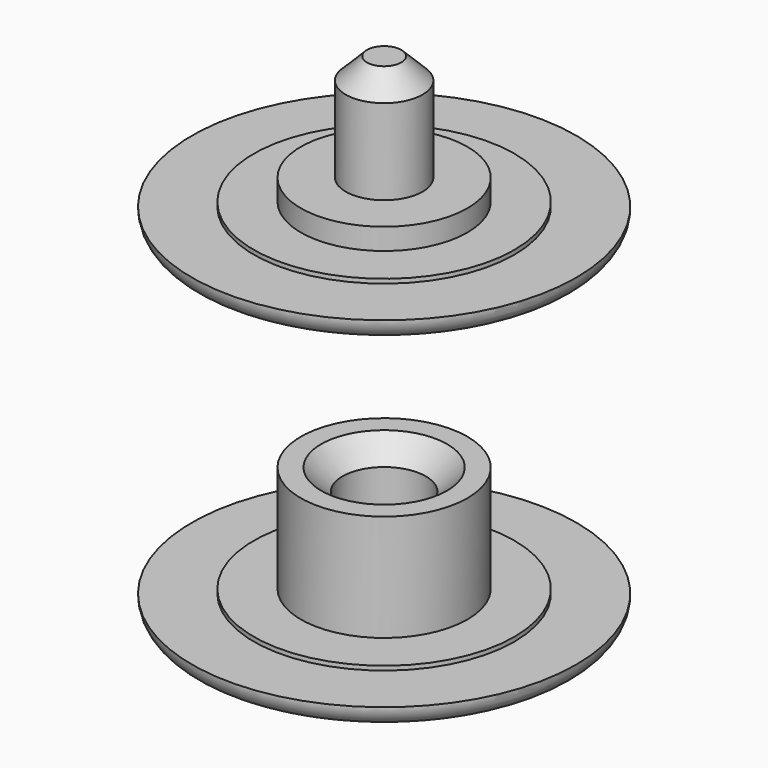
from build123d import *

# Parameters (mm, degrees)
F2_R    = 0.99999
F3_SIZE = 1
F6_R    = 0.99999
F7_SIZE = 1


# Not quite as in the source:
# - a fillet or chamfer is up to 0.001 mm smaller than in the source, because OpenCascade refuses the exact size


with BuildPart() as f1:
    # F0 (on Front) → F1 (revolve)
    with BuildSketch(Plane.XZ):
        Polygon((0, 1), (0, 0), (9, 0), (9, 1), (6.1, 1), (6.1, 1.2), (3.9, 1.2), (3.9, 6.2), (1.95, 6.2), (1.95, 2.2), (0, 2.2), (0, 1.7075754004), align=None)
    revolve(axis=Axis((0, 0, 1.9537877002), (0, 0, 1)))

    # F2 (radius 1 in the source; OpenCascade refuses exactly that, so slightly less here)
    f2_edges = [f1.edges().sort_by_distance(p)[0] for p in [
        (-9, 0, 0),
    ]]
    fillet(f2_edges, radius=F2_R)

    # F3
    f3_edges = [f1.edges().sort_by_distance(p)[0] for p in [
        (-1.95, 0, 6.2),
    ]]
    chamfer(f3_edges, length=F3_SIZE)


with BuildPart() as f5:
    # F4 (on Front) → F5 (revolve)
    with BuildSketch(Plane.XZ):
        Polygon((0, 16.9479211028), (0, 15.9479211028), (9, 15.9479211028), (9, 16.9479211028), (6.1, 16.9479211028), (6.1, 17.1479211028), (3.9, 17.1479211028), (3.9, 18.1479211028), (1.8, 18.1479211028), (1.8, 23.1479211028), (0, 23.1479211028), (0, 18.1479211028), (0, 17.1479211028), align=None)
    revolve(axis=Axis((0, 0, 17.6479211028), (0, 0, 1)))

    # F6 (radius 1 in the source; OpenCascade refuses exactly that, so slightly less here)
    f6_edges = [f5.edges().sort_by_distance(p)[0] for p in [
        (-9, 0, 15.947921),
    ]]
    fillet(f6_edges, radius=F6_R)

    # F7
    f7_edges = [f5.edges().sort_by_distance(p)[0] for p in [
        (-1.8, 0, 23.147921),
    ]]
    chamfer(f7_edges, length=F7_SIZE)


solid = Compound([f1.part, f5.part])
